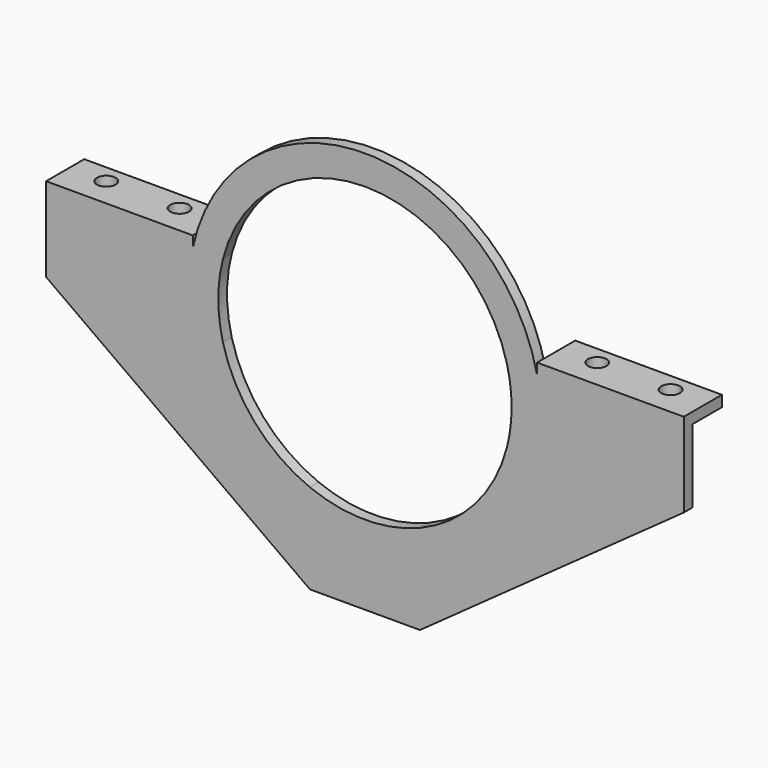
from build123d import *

# Parameters (mm, degrees)
F0_W         = 30
F0_H         = 3
F1_DEPTH     = 3
F2_W         = 40
F2_H         = 13
F2_R         = 2.55
F3_DEPTH     = 3
F4_W         = 30
F4_H         = 3
F5_DEPTH     = 25
F6_R         = 2.55
F7_DEPTH     = 3
F8_T1_DEPTH  = 30
F8_T6_DEPTH  = 20.5
F8_T11_DEPTH = 20.5
F8_T17_DEPTH = 20.5
F8_T22_DEPTH = 47.5
F8_T30_DEPTH = 20.5
F8_T35_DEPTH = 47.5


# Not quite as in the source:
# - a fillet or chamfer that OpenCascade refuses, or shapes differently, is made with other operations: its cross-section is extruded or revolved along the edge and cut away or added
# - a feature names something its author has since deleted; it is built from what else it names


with BuildPart() as f1:
    # F0 (on Front) → F1 (new body)
    with BuildSketch(Plane.XZ):
        with BuildLine():
            ThreePointArc((-46.9467783772, -10), (-48, 0), (-46.9467783772, 10))
            Line((-46.9467783772, 10), (-86.9467783772, 10))
            Line((-86.9467783772, 10), (-86.9467783772, -10))
            Line((-86.9467783772, -10), (-46.9467783772, -10))
        make_face()
        with BuildLine():
            Line((86.9467783772, 10), (46.9467783772, 10))
            ThreePointArc((46.9467783772, 10), (47.7359684206, 5.0276554125), (48, 0))
            ThreePointArc((48, 0), (47.7359684206, -5.0276554125), (46.9467783772, -10))
            Line((46.9467783772, -10), (86.9467783772, -10))
            Line((86.9467783772, -10), (86.9467783772, 10))
        make_face()
        with BuildLine():
            Line((15, -58.5960524607), (15, -45.5960524607))
            ThreePointArc((15, -45.5960524607), (0, -48), (-15, -45.5960524607))
            Line((-15, -45.5960524607), (-15, -58.5960524607))
            Line((-15, -58.5960524607), (15, -58.5960524607))
        make_face()
        with BuildLine():
            ThreePointArc((-38.7298334621, 10), (0, 40), (38.7298334621, 10))
            Line((38.7298334621, 10), (46.9467783772, 10))
            ThreePointArc((46.9467783772, 10), (0, 48), (-46.9467783772, 10))
            Line((-46.9467783772, 10), (-38.7298334621, 10))
        make_face()
        with BuildLine():
            ThreePointArc((-15, -37.0809924355), (-30.0843611996, -26.3615479669), (-38.7298334621, -10))
            Line((-38.7298334621, -10), (-46.9467783772, -10))
            ThreePointArc((-46.9467783772, -10), (-35.7228298925, -32.060558705), (-15, -45.5960524607))
            Line((-15, -45.5960524607), (-15, -37.0809924355))
        make_face()
        with BuildLine():
            Line((46.9467783772, -10), (38.7298334621, -10))
            ThreePointArc((38.7298334621, -10), (30.0843611996, -26.3615479669), (15, -37.0809924355))
            Line((15, -37.0809924355), (15, -45.5960524607))
            ThreePointArc((15, -45.5960524607), (35.7228298925, -32.060558705), (46.9467783772, -10))
        make_face()
        with BuildLine():
            ThreePointArc((-38.7298334621, -10), (-40, 0), (-38.7298334621, 10))
            Line((-38.7298334621, 10), (-46.9467783772, 10))
            ThreePointArc((-46.9467783772, 10), (-48, 0), (-46.9467783772, -10))
            Line((-46.9467783772, -10), (-38.7298334621, -10))
        make_face()
        with BuildLine():
            Line((15, -45.5960524607), (15, -37.0809924355))
            ThreePointArc((15, -37.0809924355), (0, -40), (-15, -37.0809924355))
            Line((-15, -37.0809924355), (-15, -45.5960524607))
            ThreePointArc((-15, -45.5960524607), (0, -48), (15, -45.5960524607))
        make_face()
        with BuildLine():
            ThreePointArc((38.7298334621, 10), (39.6811878507, 5.0401716993), (40, 0))
            ThreePointArc((40, 0), (39.6811878507, -5.0401716993), (38.7298334621, -10))
            Line((38.7298334621, -10), (46.9467783772, -10))
            ThreePointArc((46.9467783772, -10), (47.7359684206, -5.0276554125), (48, 0))
            ThreePointArc((48, 0), (47.7359684206, 5.0276554125), (46.9467783772, 10))
            Line((46.9467783772, 10), (38.7298334621, 10))
        make_face()
        with Locations((0, -60.0960524607)):
            Rectangle(F0_W, F0_H)
        with BuildLine():
            ThreePointArc((-15, -45.5960524607), (-35.7228298925, -32.060558705), (-46.9467783772, -10))
            Line((-46.9467783772, -10), (-86.9467783772, -10))
            Line((-86.9467783772, -10), (-15, -61.5960524607))
            Line((-15, -61.5960524607), (-15, -58.5960524607))
            Line((-15, -58.5960524607), (-15, -45.5960524607))
        make_face()
        with BuildLine():
            Line((86.9467783772, -10), (46.9467783772, -10))
            ThreePointArc((46.9467783772, -10), (35.7228298925, -32.060558705), (15, -45.5960524607))
            Line((15, -45.5960524607), (15, -58.5960524607))
            Line((15, -58.5960524607), (15, -61.5960524607))
            Line((15, -61.5960524607), (86.9467783772, -10))
        make_face()
    extrude(amount=F1_DEPTH)

    # F2 (on face) → F3 (join)
    with BuildSketch(Plane.XY.offset(10)):
        with Locations((-66.9467783772, 3.5)):
            Rectangle(F2_W, F2_H)
        with Locations((-76.9467783772, 5)):
            Circle(F2_R, mode=Mode.SUBTRACT)
        with Locations((-56.9467783772, 5)):
            Circle(F2_R, mode=Mode.SUBTRACT)
        with Locations((66.9467783772, 3.5)):
            Rectangle(F2_W, F2_H)
        with Locations((56.9467783772, 5)):
            Circle(F2_R, mode=Mode.SUBTRACT)
        with Locations((76.9467783772, 5)):
            Circle(F2_R, mode=Mode.SUBTRACT)
    extrude(amount=F3_DEPTH)

    # F4 (on face) → F5 (join)
    with BuildSketch(Plane.XZ.offset(3)):
        with Locations((0, -60.0960524607)):
            Rectangle(F4_W, F4_H)
    extrude(amount=-F5_DEPTH)

    # F6 (on face) → F7 (cut, through all)
    with BuildSketch(Plane.XY.offset(-58.5960524607)):
        with Locations((0, 12)):
            Circle(F6_R)
    extrude(amount=-F7_DEPTH, mode=Mode.SUBTRACT)

    # F8: fillet of radius 7 on 3 edges, made by hand

    # F8_s2 → F8_t1 (join)
    with BuildSketch(Plane.YZ.offset(-15)):
        with BuildLine():
            ThreePointArc((0, -51.5960524607), (2.0502525317, -56.545799929), (7, -58.5960524607))
            Line((7, -58.5960524607), (0, -58.5960524607))
            Line((0, -58.5960524607), (0, -51.5960524607))
        make_face()
    extrude(amount=F8_T1_DEPTH)


with BuildPart() as f8_tool4:
    # F8_s5 → F8_t6 (new body)
    with BuildSketch(Plane.XY.offset(-58.5960524607)):
        with BuildLine():
            ThreePointArc((-15, 7), (-17.0502525317, 2.0502525317), (-22, 0))
            Line((-22, 0), (-15, 0))
            Line((-15, 0), (-15, 7))
        make_face()
    extrude(amount=-F8_T6_DEPTH)

    split(bisect_by=Plane(origin=(-34.2651759644, 0, -47.7801867313), x_dir=(0, 1, 0), z_dir=(0.5827740813, 0, 0.8126342167)), keep=Keep.TOP)


with BuildPart() as f1_1:
    add(f1.part)

    # F8_t3: union F8_tool4
    add(f8_tool4.part)


with BuildPart() as f8_tool9:
    # F8_s10 → F8_t11 (new body)
    with BuildSketch(Plane.XY.offset(-79.0960524607)):
        with BuildLine():
            ThreePointArc((15, 7), (17.0502525317, 2.0502525317), (22, 0))
            Line((22, 0), (15, 0))
            Line((15, 0), (15, 7))
        make_face()
    extrude(amount=F8_T11_DEPTH)

    split(bisect_by=Plane(origin=(34.2651759644, 0, -47.7801867313), x_dir=(0, 1, 0), z_dir=(-0.5827740813, 0, 0.8126342167)), keep=Keep.TOP)


with BuildPart() as f1_2:
    add(f1_1.part)

    # F8_t8: union F8_tool9
    add(f8_tool9.part)


with BuildPart() as f8_tool15:
    # F8_s16 → F8_t17 (new body)
    with BuildSketch(Plane.XY.offset(-61.5960524607)):
        with BuildLine():
            ThreePointArc((15, 7), (17.0502525317, 2.0502525317), (22, 0))
            Line((22, 0), (15, 0))
            Line((15, 0), (15, 7))
        make_face()
    extrude(amount=F8_T17_DEPTH)

    split(bisect_by=Plane(origin=(34.2651759644, 0, -47.7801867313), x_dir=(0, 1, 0), z_dir=(-0.5827740813, 0, 0.8126342167)), keep=Keep.TOP)

    split(bisect_by=Plane.XY.offset(-58.5960524607), keep=Keep.TOP)


with BuildPart() as f8_tool20:
    # F8_s21 → F8_t22 (new body)
    with BuildSketch(Plane.YZ.offset(32.5)):
        with BuildLine():
            ThreePointArc((0, -51.5960524607), (2.0502525317, -56.545799929), (7, -58.5960524607))
            Line((7, -58.5960524607), (0, -58.5960524607))
            Line((0, -58.5960524607), (0, -51.5960524607))
        make_face()
    extrude(amount=-F8_T22_DEPTH)

    split(bisect_by=Plane(origin=(34.2651759644, 0, -47.7801867313), x_dir=(0, 1, 0), z_dir=(-0.5827740813, 0, 0.8126342167)), keep=Keep.TOP)

    split(bisect_by=Plane.YZ.offset(15), keep=Keep.TOP)


with BuildPart() as f8_tool15_1:
    add(f8_tool15.part)

    # F8_t25: intersect F8_tool20
    add(f8_tool20.part, mode=Mode.INTERSECT)


with BuildPart() as f1_3:
    add(f1_2.part)

    # F8_t13: union F8_tool15
    add(f8_tool15_1.part)


with BuildPart() as f8_tool28:
    # F8_s29 → F8_t30 (new body)
    with BuildSketch(Plane.XY.offset(-41.0960524607)):
        with BuildLine():
            ThreePointArc((-15, 7), (-17.0502525317, 2.0502525317), (-22, 0))
            Line((-22, 0), (-15, 0))
            Line((-15, 0), (-15, 7))
        make_face()
    extrude(amount=-F8_T30_DEPTH)

    split(bisect_by=Plane(origin=(-34.2651759644, 0, -47.7801867313), x_dir=(0, 1, 0), z_dir=(0.5827740813, 0, 0.8126342167)), keep=Keep.TOP)

    split(bisect_by=Plane.XY.offset(-58.5960524607), keep=Keep.TOP)


with BuildPart() as f8_tool33:
    # F8_s34 → F8_t35 (new body)
    with BuildSketch(Plane.YZ.offset(15)):
        with BuildLine():
            ThreePointArc((0, -51.5960524607), (2.0502525317, -56.545799929), (7, -58.5960524607))
            Line((7, -58.5960524607), (0, -58.5960524607))
            Line((0, -58.5960524607), (0, -51.5960524607))
        make_face()
    extrude(amount=-F8_T35_DEPTH)

    split(bisect_by=Plane(origin=(-34.2651759644, 0, -47.7801867313), x_dir=(0, 1, 0), z_dir=(0.5827740813, 0, 0.8126342167)), keep=Keep.TOP)

    split(bisect_by=Plane.YZ.offset(-15), keep=Keep.BOTTOM)


with BuildPart() as f8_tool28_1:
    add(f8_tool28.part)

    # F8_t38: intersect F8_tool33
    add(f8_tool33.part, mode=Mode.INTERSECT)


with BuildPart() as f1_4:
    add(f1_3.part)

    # F8_t26: union F8_tool28
    add(f8_tool28_1.part)


solid = f1_4.part
